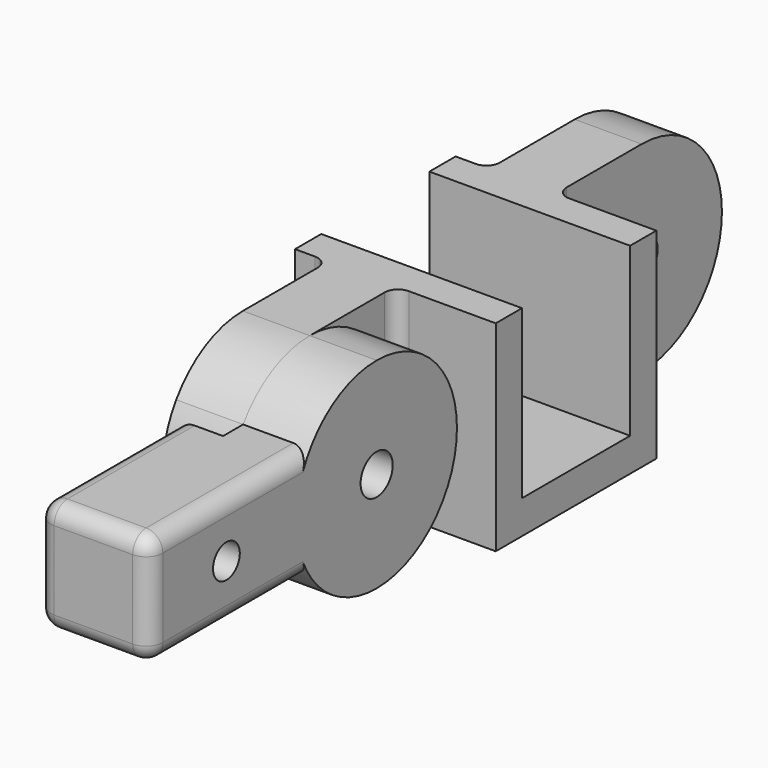
from build123d import *

# Parameters (mm, degrees)
F1_W      = 30
F1_H      = 30
F2_DEPTH  = 5
F3_W      = 30
F3_H      = 4.9
F4_DEPTH  = 25
F8_DEPTH  = 10
F9_R      = 2
F10_DEPTH = 10
F11_DEPTH = 30
F12_W     = 26.25
F12_H     = 16.75
F13_DEPTH = 6.75
F14_R     = 3
F15_DEPTH = 25
F16_R     = 2.5
F17_R     = 2.5
F18_DEPTH = 16.75


with BuildPart() as f2:
    # F1 (on Top) → F2 (new body)
    with BuildSketch(Plane.XY):
        with Locations((15, 15)):
            Rectangle(F1_W, F1_H)
    extrude(amount=F2_DEPTH)

    # F3 (on face) → F4 (join)
    with BuildSketch(Plane.XY.offset(5)):
        with Locations((15, 27.55)):
            Rectangle(F3_W, F3_H)
        with Locations((15, 2.45)):
            Rectangle(F3_W, F3_H)
    extrude(amount=F4_DEPTH)

    # F7 (on line) → F8 (join)
    with BuildSketch(Plane(origin=(15, 0, 0), x_dir=(0, -1, 0), z_dir=(-1, 0, 0))):
        with BuildLine():
            Line((16, 30), (0, 30))
            Line((0, 30), (0, 0))
            Line((0, 0), (16, 0))
            ThreePointArc((16, 0), (1, 15), (16, 30))
        make_face()
        with BuildLine():
            ThreePointArc((28.4442506805, 23.375), (23.0489360899, 28.2405626769), (16, 30))
            Line((16, 30), (16, 23))
            Line((16, 23), (16, 7))
            Line((16, 7), (16, 0))
            ThreePointArc((16, 0), (23.0489360899, 1.7594373231), (28.4442506805, 6.625))
            Line((28.4442506805, 6.625), (28.4442506805, 23.375))
        make_face()
        with BuildLine():
            Line((16, 23), (16, 30))
            ThreePointArc((16, 30), (1, 15), (16, 0))
            Line((16, 0), (16, 7))
            Line((16, 7), (16, 23))
        make_face()
        with BuildLine():
            ThreePointArc((31, 15), (30.3468421649, 19.3781411462), (28.4442506805, 23.375))
            Line((28.4442506805, 23.375), (28.4442506805, 6.625))
            ThreePointArc((28.4442506805, 6.625), (30.3468421649, 10.6218588538), (31, 15))
        make_face()
        with BuildLine():
            Line((-46, 0), (-46, 30))
            ThreePointArc((-46, 30), (-53.0489360899, 28.2405626769), (-58.4442506805, 23.375))
            Line((-58.4442506805, 23.375), (-58.4442506805, 6.625))
            ThreePointArc((-58.4442506805, 6.625), (-53.0489360899, 1.7594373231), (-46, 0))
        make_face()
        with BuildLine():
            ThreePointArc((-31, 15), (-35.3933982822, 25.6066017178), (-46, 30))
            Line((-46, 30), (-46, 0))
            ThreePointArc((-46, 0), (-35.3933982822, 4.3933982822), (-31, 15))
        make_face()
        with BuildLine():
            Line((-30, 0), (-30, 30))
            Line((-30, 30), (-46, 30))
            ThreePointArc((-46, 30), (-35.3933982822, 25.6066017178), (-31, 15))
            ThreePointArc((-31, 15), (-35.3933982822, 4.3933982822), (-46, 0))
            Line((-46, 0), (-30, 0))
        make_face()
        with BuildLine():
            Line((-58.4442506805, 6.625), (-58.4442506805, 23.375))
            ThreePointArc((-58.4442506805, 23.375), (-61, 15), (-58.4442506805, 6.625))
        make_face()
    extrude(amount=F8_DEPTH)

    # F9
    f9_edges = [f2.edges().sort_by_distance(p)[0] for p in [
        (5, 0, 15),
        (15, 0, 15),
        (5, 30, 15),
        (15, 30, 15),
    ]]
    fillet(f9_edges, radius=F9_R)


with BuildPart() as f10:
    # F7 (on line) → F10 (new body)
    with BuildSketch(Plane(origin=(15, 0, 0), x_dir=(0, -1, 0), z_dir=(-1, 0, 0))):
        with BuildLine():
            Line((16, 23), (16, 30))
            ThreePointArc((16, 30), (1, 15), (16, 0))
            Line((16, 0), (16, 7))
            Line((16, 7), (16, 23))
        make_face()
        with BuildLine():
            ThreePointArc((28.4442506805, 23.375), (23.0489360899, 28.2405626769), (16, 30))
            Line((16, 30), (16, 23))
            Line((16, 23), (16, 7))
            Line((16, 7), (16, 0))
            ThreePointArc((16, 0), (23.0489360899, 1.7594373231), (28.4442506805, 6.625))
            Line((28.4442506805, 6.625), (28.4442506805, 23.375))
        make_face()
    extrude(amount=-F10_DEPTH)

    # F11 (add): a face of the model
    f11_faces = [f10.faces().sort_by_distance(p)[0] for p in [
        (20, -28.4442506805, 15),
    ]]
    extrude(f11_faces, amount=F11_DEPTH)

    # F12 (on face) → F13 (join)
    with BuildSketch(Plane(origin=(15, 0, 0), x_dir=(0, -1, 0), z_dir=(-1, 0, 0))):
        with Locations((45.3192506805, 15)):
            Rectangle(F12_W, F12_H)
    extrude(amount=F13_DEPTH)


with BuildPart() as f15_tool:
    # F14 (on face) → F15 (new body)
    with BuildSketch(Plane.YZ.offset(25)):
        with Locations((-16, 15)):
            Circle(F14_R)
        with Locations((46, 15)):
            Circle(F14_R)
    extrude(amount=-F15_DEPTH)


with BuildPart() as f2_1:
    add(f2.part)

    # F15: cut by f15_tool
    add(f15_tool.part, mode=Mode.SUBTRACT)


with BuildPart() as f10_1:
    add(f10.part)

    # F15: cut by f15_tool
    add(f15_tool.part, mode=Mode.SUBTRACT)

    # F16
    f16_edges = [f10_1.edges().sort_by_distance(p)[0] for p in [
        (8.25, -45.319251, 23.375),
        (8.25, -45.319251, 6.625),
        (25, -43.444251, 23.375),
        (25, -43.444251, 6.625),
        (25, -58.444251, 15),
        (8.25, -58.444251, 15),
        (16.625, -58.444251, 6.625),
        (16.625, -58.444251, 23.375),
    ]]
    fillet(f16_edges, radius=F16_R)

    # F17 (on face) → F18 (cut, through all)
    with BuildSketch(Plane(origin=(8.25, 0, 0), x_dir=(0, -1, 0), z_dir=(-1, 0, 0))):
        with Locations((44.0692506805, 15)):
            Circle(F17_R)
    extrude(amount=-F18_DEPTH, mode=Mode.SUBTRACT)


solid = Compound([f2_1.part, f10_1.part])
